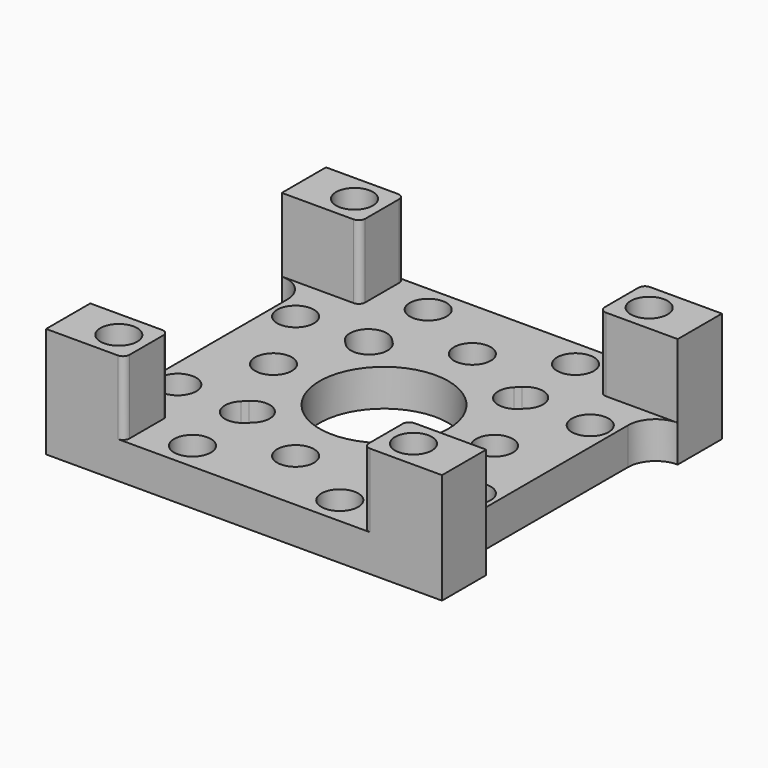
from build123d import *

# Parameters (mm, degrees)
F0_W     = 43
F0_H     = 38
F0_R     = 2
F0_R_2   = 7
F1_DEPTH = 4
F2_W     = 8.5
F2_H     = 6
F2_R     = 2
F3_DEPTH = 8
F4_W     = 3
F4_H     = 26
F5_DEPTH = 25
F6_R     = 2.99999
F7_R     = 0.7


# Not quite as in the source:
# - a fillet or chamfer is up to 0.001 mm smaller than in the source, because OpenCascade refuses the exact size


with BuildPart() as f1:
    # F0 (on Top) → F1 (new body)
    with BuildSketch(Plane.XY):
        Rectangle(F0_W, F0_H)
        with Locations((-16, -16)):
            Circle(F0_R, mode=Mode.SUBTRACT)
        with Locations((-8, -16)):
            Circle(F0_R, mode=Mode.SUBTRACT)
        with Locations((-16, -8)):
            Circle(F0_R, mode=Mode.SUBTRACT)
        with BuildLine():
            ThreePointArc((-9.4142135624, -6.5857864376), (-6.5857864376, -6.5857864376), (-6.5857864376, -9.4142135624))
            Line((-6.5857864376, -9.4142135624), (-7.0710678119, -9.8994949366))
            ThreePointArc((-7.0710678119, -9.8994949366), (-9.8994949366, -9.8994949366), (-9.8994949366, -7.0710678119))
            Line((-9.8994949366, -7.0710678119), (-9.4142135624, -6.5857864376))
        make_face(mode=Mode.SUBTRACT)
        with Locations((8, -16)):
            Circle(F0_R, mode=Mode.SUBTRACT)
        with Locations((0, -12)):
            Circle(F0_R, mode=Mode.SUBTRACT)
        with Locations((16, -16)):
            Circle(F0_R, mode=Mode.SUBTRACT)
        with BuildLine():
            ThreePointArc((6.5857864376, -9.4142135624), (6.5857864376, -6.5857864376), (9.4142135624, -6.5857864376))
            Line((9.4142135624, -6.5857864376), (9.8994949366, -7.0710678119))
            ThreePointArc((9.8994949366, -7.0710678119), (9.8994949366, -9.8994949366), (7.0710678119, -9.8994949366))
            Line((7.0710678119, -9.8994949366), (6.5857864376, -9.4142135624))
        make_face(mode=Mode.SUBTRACT)
        with Locations((16, -8)):
            Circle(F0_R, mode=Mode.SUBTRACT)
        with Locations((-12, 0)):
            Circle(F0_R, mode=Mode.SUBTRACT)
        with Locations((-16, 8)):
            Circle(F0_R, mode=Mode.SUBTRACT)
        with BuildLine():
            ThreePointArc((-6.5857864376, 9.4142135624), (-6.5857864376, 6.5857864376), (-9.4142135624, 6.5857864376))
            Line((-9.4142135624, 6.5857864376), (-9.8994949366, 7.0710678119))
            ThreePointArc((-9.8994949366, 7.0710678119), (-9.8994949366, 9.8994949366), (-7.0710678119, 9.8994949366))
            Line((-7.0710678119, 9.8994949366), (-6.5857864376, 9.4142135624))
        make_face(mode=Mode.SUBTRACT)
        with Locations((-16, 16)):
            Circle(F0_R, mode=Mode.SUBTRACT)
        with Locations((-8, 16)):
            Circle(F0_R, mode=Mode.SUBTRACT)
        Circle(F0_R_2, mode=Mode.SUBTRACT)
        with BuildLine():
            ThreePointArc((9.4142135624, 6.5857864376), (6.5857864376, 6.5857864376), (6.5857864376, 9.4142135624))
            Line((6.5857864376, 9.4142135624), (7.0710678119, 9.8994949366))
            ThreePointArc((7.0710678119, 9.8994949366), (9.8994949366, 9.8994949366), (9.8994949366, 7.0710678119))
            Line((9.8994949366, 7.0710678119), (9.4142135624, 6.5857864376))
        make_face(mode=Mode.SUBTRACT)
        with Locations((12, 0)):
            Circle(F0_R, mode=Mode.SUBTRACT)
        with Locations((16, 8)):
            Circle(F0_R, mode=Mode.SUBTRACT)
        with Locations((0, 12)):
            Circle(F0_R, mode=Mode.SUBTRACT)
        with Locations((8, 16)):
            Circle(F0_R, mode=Mode.SUBTRACT)
        with Locations((16, 16)):
            Circle(F0_R, mode=Mode.SUBTRACT)
    extrude(amount=F1_DEPTH)

    # F2 (on face) → F3 (join)
    with BuildSketch(Plane.XY.offset(4)):
        with Locations((-17.25, 16)):
            Rectangle(F2_W, F2_H)
        with Locations((-16, 16)):
            Circle(F2_R, mode=Mode.SUBTRACT)
        with Locations((17.25, 16)):
            Rectangle(F2_W, F2_H)
        with Locations((16, 16)):
            Circle(F2_R, mode=Mode.SUBTRACT)
        with Locations((17.25, -16)):
            Rectangle(F2_W, F2_H)
        with Locations((16, -16)):
            Circle(F2_R, mode=Mode.SUBTRACT)
        with Locations((-17.25, -16)):
            Rectangle(F2_W, F2_H)
        with Locations((-16, -16)):
            Circle(F2_R, mode=Mode.SUBTRACT)
    extrude(amount=F3_DEPTH)

    # F4 (on face) → F5 (cut)
    with BuildSketch(Plane.XY.offset(4)):
        with Locations((-20, 0)):
            Rectangle(F4_W, F4_H)
        with Locations((20, 0)):
            Rectangle(F4_W, F4_H)
    extrude(amount=-F5_DEPTH, mode=Mode.SUBTRACT)

    # F6 (radius 3 in the source; OpenCascade refuses exactly that, so slightly less here)
    f6_edges = [f1.edges().sort_by_distance(p)[0] for p in [
        (-18.5, 13, 2),
        (-18.5, -13, 2),
        (18.5, 13, 2),
        (18.5, -13, 2),
    ]]
    fillet(f6_edges, radius=F6_R)

    # F7
    f7_edges = [f1.edges().sort_by_distance(p)[0] for p in [
        (13, 13, 8),
        (13, -19, 8),
        (13, -13, 8),
        (-13, -19, 8),
        (-13, 13, 8),
        (-13, 19, 8),
        (-13, -13, 8),
        (13, 19, 8),
    ]]
    fillet(f7_edges, radius=F7_R)


solid = f1.part
